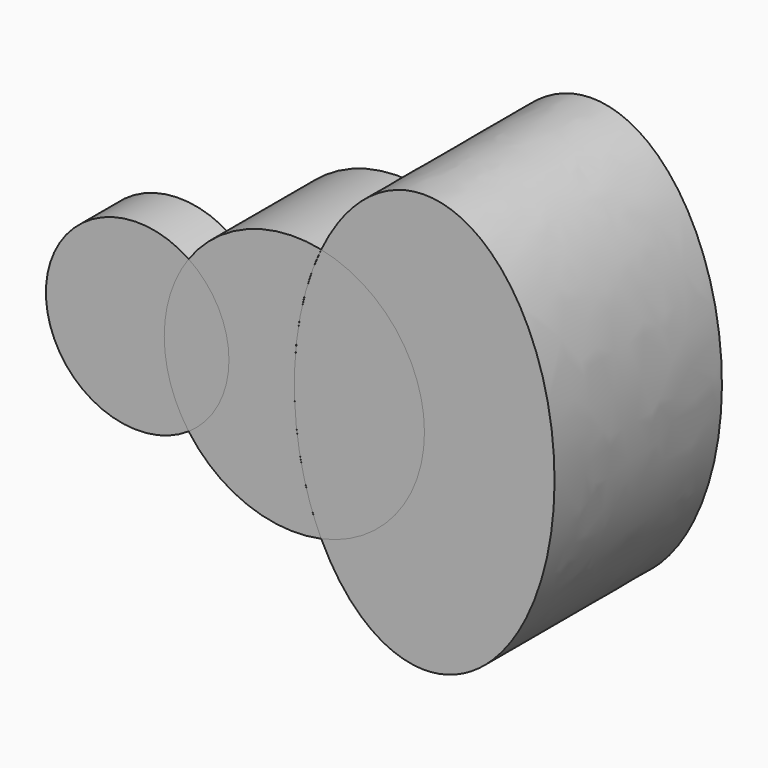
from build123d import *

# Parameters (mm, degrees)
F1_DEPTH = 63.5
F2_DEPTH = 101.6
F3_DEPTH = 25.4
F4_DEPTH = 63.5
F5_DEPTH = 101.6


# Not quite as in the source:
# - a feature names something its author has since deleted; it is built from what else it names


with BuildPart() as f1:
    # F0 (on Front) → F1 (new body)
    with BuildSketch(Plane.XZ):
        with BuildLine():
            add(Edge.make_bspline(
                [(0, 0), (0, -34.4673908513), (13.0417227804, -61.8200466708)],
                knots=[4.7123889804, 4.7123889804, 4.7123889804, 5.366513896, 5.366513896, 5.366513896], degree=2, weights=[1, 0.9469901505, 1]))
            Line((0, 0), (-31.75, 0))
            ThreePointArc((-31.75, 0), (-36.9485869215, -20.8597476336), (-51.3283609151, -36.8402506673))
            ThreePointArc((-51.3283609151, -36.8402506673), (-22.8574761732, -58.9011076844), (13.0417227804, -61.8200466708))
        make_face()
        with BuildLine():
            Line((-31.75, 0), (0, 0))
            add(Edge.make_bspline(
                [(13.0417227804, 61.8200466708), (0, 34.4673908513), (0, 0)],
                knots=[4.0582640648, 4.0582640648, 4.0582640648, 4.7123889804, 4.7123889804, 4.7123889804], degree=2, weights=[1, 0.9469901505, 1]))
            ThreePointArc((13.0417227804, 61.8200466708), (-22.8574761732, 58.9011076844), (-51.3283609151, 36.8402506673))
            ThreePointArc((-51.3283609151, 36.8402506673), (-36.9485869215, 20.8597476336), (-31.75, 0))
        make_face()
    extrude(amount=-F1_DEPTH)


with BuildPart() as f2:
    # F0 (on Front) → F2 (new body)
    with BuildSketch(Plane.XZ):
        with BuildLine():
            ThreePointArc((63.1807304759, 0), (49.0703081068, -39.7983613452), (13.0417227804, -61.8200466708))
            add(Edge.make_bspline(
                [(13.0417227804, -61.8200466708), (74.8763980172, -191.5070993665), (119.8405851231, -44.9535496832), (164.804772229, 101.6), (63.1807304759, 101.6)],
                knots=[5.366513896, 5.366513896, 5.366513896, 7.3956459284, 7.3956459284, 9.4247779608, 9.4247779608, 9.4247779608], degree=2, weights=[1, 0.5279885426, 1, 0.5279885426, 1]))
            Line((63.1807304759, 101.6), (63.1807304759, 0))
        make_face()
        with BuildLine():
            add(Edge.make_bspline(
                [(63.1807304759, 101.6), (32.00877033, 101.6), (13.0417227804, 61.8200466708)],
                knots=[3.1415926536, 3.1415926536, 3.1415926536, 4.0582640648, 4.0582640648, 4.0582640648], degree=2, weights=[1, 0.8967901166, 1]))
            ThreePointArc((13.0417227804, 61.8200466708), (49.0703081068, 39.7983613452), (63.1807304759, 0))
            Line((63.1807304759, 0), (63.1807304759, 101.6))
        make_face()
    extrude(amount=-F2_DEPTH)


with BuildPart() as f3:
    # F0 (on Front) → F3 (new body)
    with BuildSketch(Plane.XZ):
        with BuildLine():
            add(Edge.make_bspline(
                [(13.0417227804, 61.8200466708), (0, 34.4673908513), (0, 0)],
                knots=[4.0582640648, 4.0582640648, 4.0582640648, 4.7123889804, 4.7123889804, 4.7123889804], degree=2, weights=[1, 0.9469901505, 1]))
            add(Edge.make_bspline(
                [(0, 0), (0, -34.4673908513), (13.0417227804, -61.8200466708)],
                knots=[4.7123889804, 4.7123889804, 4.7123889804, 5.366513896, 5.366513896, 5.366513896], degree=2, weights=[1, 0.9469901505, 1]))
            ThreePointArc((13.0417227804, -61.8200466708), (49.0703081068, -39.7983613452), (63.1807304759, 0))
            ThreePointArc((63.1807304759, 0), (49.0703081068, 39.7983613452), (13.0417227804, 61.8200466708))
        make_face()
    extrude(amount=-F3_DEPTH)

    # F0 (on Front) → F5 (join)
    with BuildSketch(Plane.XZ):
        with BuildLine():
            add(Edge.make_bspline(
                [(13.0417227804, 61.8200466708), (0, 34.4673908513), (0, 0)],
                knots=[4.0582640648, 4.0582640648, 4.0582640648, 4.7123889804, 4.7123889804, 4.7123889804], degree=2, weights=[1, 0.9469901505, 1]))
            add(Edge.make_bspline(
                [(0, 0), (0, -34.4673908513), (13.0417227804, -61.8200466708)],
                knots=[4.7123889804, 4.7123889804, 4.7123889804, 5.366513896, 5.366513896, 5.366513896], degree=2, weights=[1, 0.9469901505, 1]))
            ThreePointArc((13.0417227804, -61.8200466708), (49.0703081068, -39.7983613452), (63.1807304759, 0))
            ThreePointArc((63.1807304759, 0), (49.0703081068, 39.7983613452), (13.0417227804, 61.8200466708))
        make_face()
    extrude(amount=-F5_DEPTH)


with BuildPart() as f3b:
    # F0 (on Front) → F3, piece 2 (new body)
    with BuildSketch(Plane.XZ):
        with BuildLine():
            ThreePointArc((-51.3283609151, -36.8402506673), (-60.1446923685, -19.3499530583), (-63.1807304759, 0))
            ThreePointArc((-63.1807304759, 0), (-60.1446923685, 19.3499530583), (-51.3283609151, 36.8402506673))
            ThreePointArc((-51.3283609151, 36.8402506673), (-120.65, 0), (-51.3283609151, -36.8402506673))
        make_face()
    extrude(amount=-F3_DEPTH)


with BuildPart() as f4:
    # F0 (on Front) → F4 (new body)
    with BuildSketch(Plane.XZ):
        with BuildLine():
            ThreePointArc((-51.3283609151, -36.8402506673), (-36.9485869215, -20.8597476336), (-31.75, 0))
            Line((-31.75, 0), (-63.1807304759, 0))
            ThreePointArc((-63.1807304759, 0), (-60.1446923685, -19.3499530583), (-51.3283609151, -36.8402506673))
        make_face()
        with BuildLine():
            Line((-63.1807304759, 0), (-31.75, 0))
            ThreePointArc((-31.75, 0), (-36.9485869215, 20.8597476336), (-51.3283609151, 36.8402506673))
            ThreePointArc((-51.3283609151, 36.8402506673), (-60.1446923685, 19.3499530583), (-63.1807304759, 0))
        make_face()
    extrude(amount=-F4_DEPTH)


solid = Compound([f1.part, f2.part, f3.part, f3b.part, f4.part])
